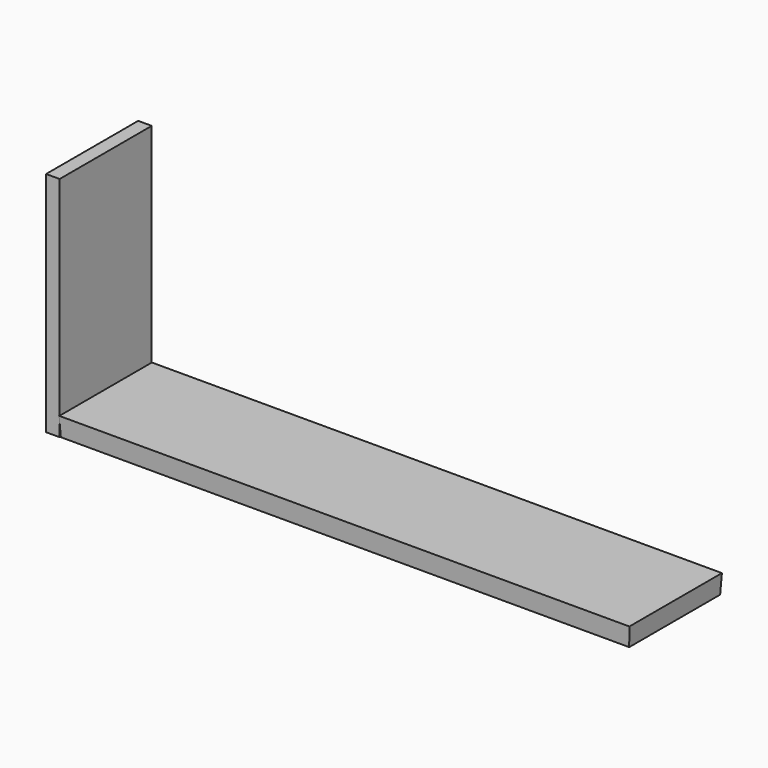
from build123d import *

# Parameters (mm, degrees)
F0_W      = 1524
F0_H      = 304.8
F1_DEPTH  = 25.4
F1_TAPER  = -3
F1_FACE_W = 1526.6623151876
F1_FACE_H = 307.4623151876
F3_DEPTH  = 25.4
F3_TAPER  = -3
F4_W      = 36.3832712173
F4_H      = 308.6890354753
F5_DEPTH  = 609.6


# Not quite as in the source:
# - a feature names something its author has since deleted; it is built from what else it names


with BuildPart() as f1:
    # F0 (on Top) → F1 (new body)
    with BuildSketch(Plane.XY):
        with Locations((-1.6607679427, -79.0239475151)):
            Rectangle(F0_W, F0_H)
    extrude(amount=F1_DEPTH, taper=F1_TAPER)

    # F1_face (on face) → F3 (join)
    with BuildSketch(Plane(origin=(-1.6607679427, -79.0239475151, 25.4), x_dir=(1, 0, 0), z_dir=(0, 0, 1))):
        Rectangle(F1_FACE_W, F1_FACE_H)
    extrude(amount=F3_DEPTH, taper=F3_TAPER)

    # F4 (on Top) → F5 (join)
    with BuildSketch(Plane.XY):
        with Locations((-783.7679982185, -78.7090621889)):
            Rectangle(F4_W, F4_H)
    extrude(amount=F5_DEPTH)


solid = f1.part
